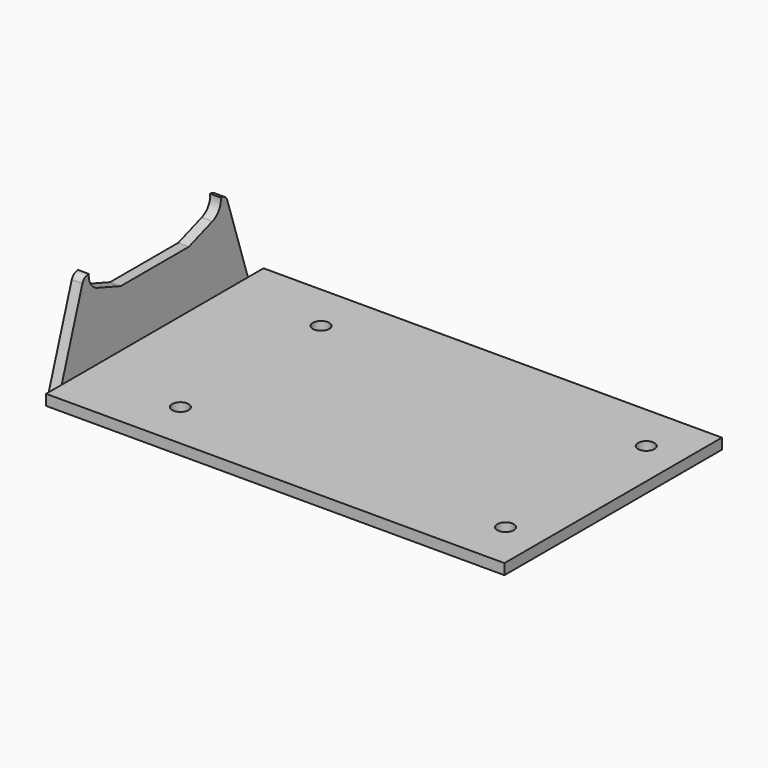
from build123d import *

# Parameters (mm, degrees)
F0_W        = 86
F0_H        = 51
F1_DEPTH    = 2
F3_R        = 1.55
F4_DEPTH    = 25.4
F5_DEPTH    = 2
F6_T1_DEPTH = 9.0710678119


# Not quite as in the source:
# - a fillet or chamfer that OpenCascade refuses, or shapes differently, is made with other operations: its cross-section is extruded or revolved along the edge and cut away or added


with BuildPart() as f1:
    # F0 (on Top) → F1 (new body)
    with BuildSketch(Plane.XY):
        Rectangle(F0_W, F0_H)
    extrude(amount=F1_DEPTH)

    # F3 (on face) → F4 (cut)
    with BuildSketch(Plane.XY.offset(2)):
        with Locations((-25, 16.5)):
            Circle(F3_R)
        with Locations((-25, -16.5)):
            Circle(F3_R)
        with Locations((36, 16.5)):
            Circle(F3_R)
        with Locations((36, -16.5)):
            Circle(F3_R)
    extrude(amount=-F4_DEPTH, mode=Mode.SUBTRACT)

    # F2 (on face) → F5 (join)
    with BuildSketch(Plane(origin=(-43, 0, 0), x_dir=(0, -1, 0), z_dir=(-1, 0, 0))):
        with BuildLine():
            Line((8, 12.6704787835), (0, 12.6704787835))
            Line((0, 12.6704787835), (-8, 12.6704787835))
            Line((-8, 12.6704787835), (-13.5029918403, 14.6226324313))
            ThreePointArc((-13.5029918403, 14.6226324313), (-15.0300310094, 15.8378762171), (-15.4863987014, 17.7353468))
            Line((-15.4863987014, 17.7353468), (-16.9863987014, 17.7353468))
            Line((-16.9863987014, 17.7353468), (-16.9863987014, 16.7353468))
            Line((-16.9863987014, 16.7353468), (-22.5, 0))
            Line((-22.5, 0), (22.5, 0))
            Line((22.5, 0), (16.9863987014, 16.7353468))
            Line((16.9863987014, 16.7353468), (16.9863987014, 17.7353468))
            Line((16.9863987014, 17.7353468), (15.4863987014, 17.7353468))
            ThreePointArc((15.4863987014, 17.7353468), (15.0300310094, 15.8378762171), (13.5029918403, 14.6226324313))
            Line((13.5029918403, 14.6226324313), (8, 12.6704787835))
        make_face()
        with BuildLine():
            Line((8, 12.6704787835), (0, 12.6704787835))
            Line((0, 12.6704787835), (-8, 12.6704787835))
            Line((-8, 12.6704787835), (-13.5029918403, 14.6226324313))
            ThreePointArc((-13.5029918403, 14.6226324313), (-15.0300310094, 15.8378762171), (-15.4863987014, 17.7353468))
            Line((-15.4863987014, 17.7353468), (-16.9863987014, 17.7353468))
            Line((-16.9863987014, 17.7353468), (-16.9863987014, 16.7353468))
            Line((-16.9863987014, 16.7353468), (-21.8410831141, 2))
            Line((-21.8410831141, 2), (21.8410831141, 2))
            Line((21.8410831141, 2), (16.9863987014, 16.7353468))
            Line((16.9863987014, 16.7353468), (16.9863987014, 17.7353468))
            Line((16.9863987014, 17.7353468), (15.4863987014, 17.7353468))
            ThreePointArc((15.4863987014, 17.7353468), (15.0300310094, 15.8378762171), (13.5029918403, 14.6226324313))
            Line((13.5029918403, 14.6226324313), (8, 12.6704787835))
        make_face()
    extrude(amount=F5_DEPTH)

    # F6: fillet of radius 1.5 on 2 edges, made by hand

    # F6_s2 → F6_t1 (cut)
    with BuildSketch(Plane.YZ.offset(-48.5355339059)):
        with BuildLine():
            ThreePointArc((-15.572185139, 17.7353468), (-16.4382105428, 17.4600916714), (-16.9863987014, 16.7353468))
            Line((-16.9863987014, 16.7353468), (-16.9863987014, 17.7353468))
            Line((-16.9863987014, 17.7353468), (-15.572185139, 17.7353468))
        make_face()
        with BuildLine():
            ThreePointArc((16.9863987014, 16.7353468), (16.4382105428, 17.4600916714), (15.572185139, 17.7353468))
            Line((15.572185139, 17.7353468), (16.9863987014, 17.7353468))
            Line((16.9863987014, 17.7353468), (16.9863987014, 16.7353468))
        make_face()
    extrude(amount=F6_T1_DEPTH, mode=Mode.SUBTRACT)


solid = f1.part
